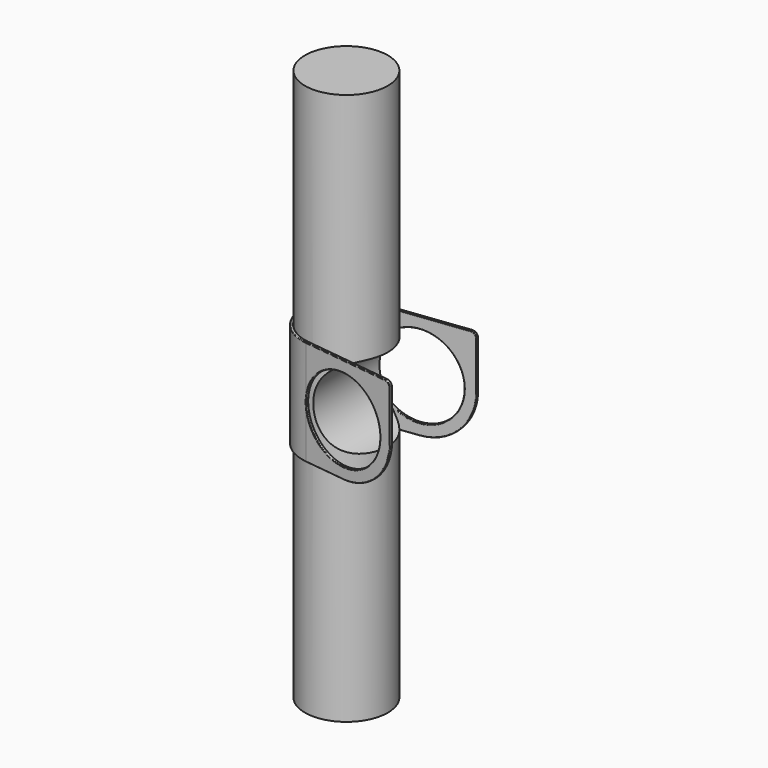
from build123d import *

# Parameters (mm, degrees)
F1_DEPTH  = 19
F2_R      = 19
F3_R      = 2
F4_R      = 0.2
F5_R      = 15
F6_DEPTH  = 1
F7_R      = 0.2
F8_R      = 15
F9_DEPTH  = 100
F10_R     = 15
F11_DEPTH = 20


# Not quite as in the source:
# - a pattern or mirror of a feature is missing from the dataset's text; its kind, count and spacing are read off the source's solid


with BuildPart() as f1:
    # F0 (on Top) → F1 (new body, symmetric)
    with BuildSketch(Plane.XY):
        with BuildLine():
            ThreePointArc((-21.8280401511, -14.8881922746), (-35, 0), (-21.8280401511, 14.8881922746))
            Line((-21.8280401511, 14.8881922746), (11.9185290047, 19.0317499504))
            Line((11.9185290047, 19.0317499504), (11.7966596613, 20.024296102))
            Line((11.7966596613, 20.024296102), (-21.9499094945, 15.8807384263))
            ThreePointArc((-21.9499094945, 15.8807384263), (-36, 0), (-21.9499094945, -15.8807384263))
            Line((-21.9499094945, -15.8807384263), (11.7966596613, -20.024296102))
            Line((11.7966596613, -20.024296102), (11.9185290047, -19.0317499504))
            Line((11.9185290047, -19.0317499504), (-21.8280401511, -14.8881922746))
        make_face()
    extrude(amount=F1_DEPTH, both=True)

    # F2
    f2_edges = [f1.edges().sort_by_distance(p)[0] for p in [
        (11.857594, 19.528023, -19),
        (11.857594, -19.528023, -19),
    ]]
    fillet(f2_edges, radius=F2_R)

    # F3
    f3_edges = [f1.edges().sort_by_distance(p)[0] for p in [
        (11.857594, -19.528023, 19),
        (11.857594, 19.528023, 19),
    ]]
    fillet(f3_edges, radius=F3_R)

    # F4
    f4_edges = [f1.edges().sort_by_distance(p)[0] for p in [
        (11.79666, -20.024296, 8.5),
        (11.337109, -18.960361, 18.414214),
    ]]
    fillet(f4_edges, radius=F4_R)

    # F5 (on face) → F6 (cut)
    with BuildSketch(Plane(origin=(-2.2469522317, -18.2999573823, 0), x_dir=(0.9925461516, -0.1218693434, 0), z_dir=(-0.1218693434, -0.9925461516, 0))):
        with Locations((-4.8509230328, 0)):
            Circle(F5_R)
    f6 = extrude(amount=-F6_DEPTH, mode=Mode.SUBTRACT)

    # F6_copies: F6 across plane
    add(f6.mirror(Plane.ZX), mode=Mode.SUBTRACT)

    # F7
    f7_edges = [f1.edges().sort_by_distance(p)[0] for p in [
        (-7.061717, -17.708779, 15),
        (-7.061717, -17.708779, -15),
        (7.88741, -19.040546, 0),
        (-6.939848, -16.716232, -15),
        (-6.939848, -16.716232, 15),
        (-7.061717, 17.708779, 15),
        (-7.061717, 17.708779, -15),
        (-6.939848, 16.716232, -15),
        (-6.939848, 16.716232, 15),
    ]]
    fillet(f7_edges, radius=F7_R)


with BuildPart() as f9:
    # F8 (on Top) → F9 (new body, symmetric)
    with BuildSketch(Plane.XY):
        with Locations((-20, 0)):
            Circle(F8_R)
    extrude(amount=F9_DEPTH, both=True)

    # F10 (on Front) → F11 (cut, symmetric)
    with BuildSketch(Plane.XZ):
        with Locations((-5.0069657154, 0)):
            Circle(F10_R)
    extrude(amount=F11_DEPTH, both=True, mode=Mode.SUBTRACT)


solid = Compound([f1.part, f9.part])
